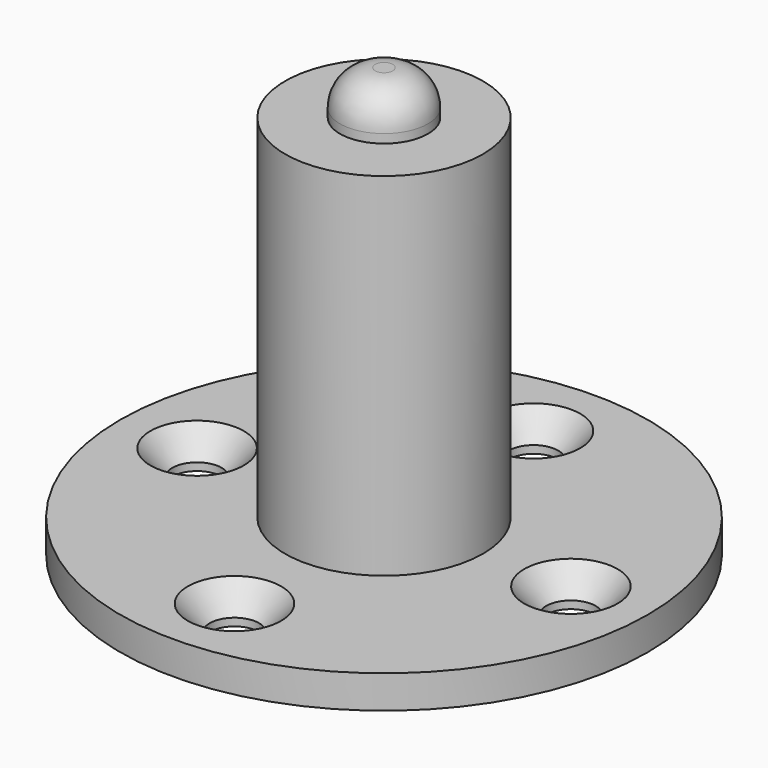
from build123d import *

# Parameters (mm, degrees)
F0_R            = 38.1
F1_DEPTH        = 4.7625
F2_R            = 14.2875
F3_DEPTH        = 50.8
F4_R            = 6.35
F5_DEPTH        = 6.35
F6_R            = 5.08
F8_D            = 7.1374
F8_DEPTH        = 15.875
F8_CSINK_D      = 13.4874
F8_CSINK_ANGLE  = 82
F8_TIP          = 2.1442912911
F8_COPIES_COUNT = 4


# Not quite as in the source:
# - a pattern or mirror of a feature is missing from the dataset's text; its kind, count and spacing are read off the source's solid


with BuildPart() as f1:
    # F0 (on Top) → F1 (new body)
    with BuildSketch(Plane.XY):
        Circle(F0_R)
    extrude(amount=F1_DEPTH)

    # F2 (on face) → F3 (join)
    with BuildSketch(Plane.XY.offset(4.7625)):
        Circle(F2_R)
    extrude(amount=F3_DEPTH)

    # F4 (on face) → F5 (join)
    with BuildSketch(Plane.XY.offset(55.5625)):
        Circle(F4_R)
    extrude(amount=F5_DEPTH)

    # F6
    f6_edges = [f1.edges().sort_by_distance(p)[0] for p in [
        (-6.35, 0, 61.9125),
    ]]
    fillet(f6_edges, radius=F6_R)

    # F8
    with Locations(Plane.XY.offset(4.7625)):
        with Locations((0, -26.9875)):
            f8 = CounterSinkHole(F8_D / 2, F8_CSINK_D / 2, depth=F8_DEPTH, counter_sink_angle=F8_CSINK_ANGLE)
            with Locations((0, 0, -(F8_DEPTH + F8_TIP / 2))):  # 118° drill point
                Cone(0, F8_D / 2, F8_TIP, mode=Mode.SUBTRACT)

    # F8_copies: F8 ×4 about axis
    f8_copies_axis = Axis((0, 0, 0), (0, 0, 1))
    for i in range(1, F8_COPIES_COUNT):
        add(f8.rotate(f8_copies_axis, i * 360 / F8_COPIES_COUNT), mode=Mode.SUBTRACT)


solid = f1.part
